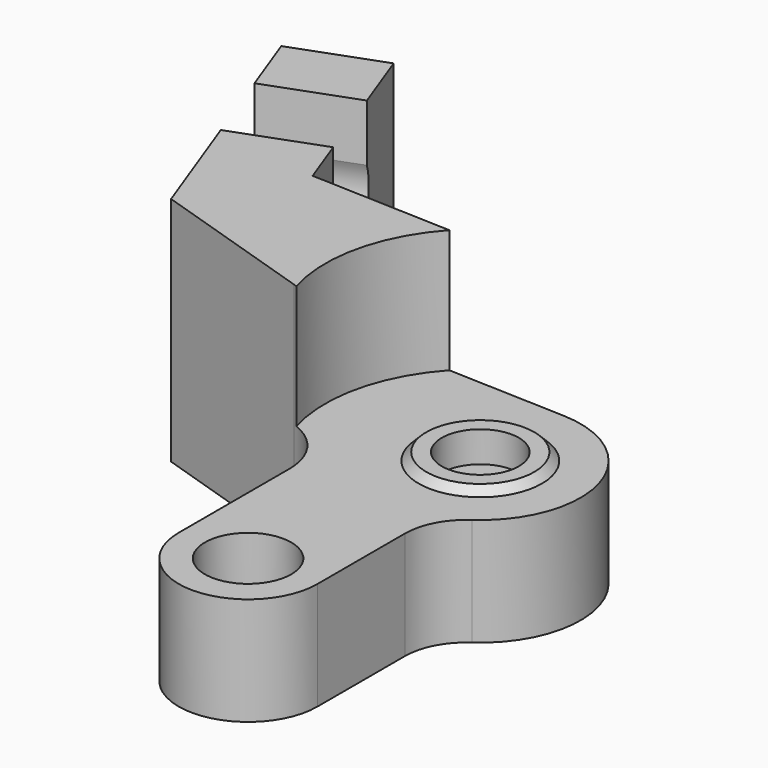
from build123d import *

# Parameters (mm, degrees)
F1_DEPTH       = 15
F3_DEPTH       = 8
F5_D           = 3.2
F5_CBORE_D     = 5.6
F5_CBORE_DEPTH = 3
F6_R           = 4.5
F7_DEPTH       = 5
F8_R           = 4
F9_DEPTH       = 0.5
F10_R          = 2.5
F11_DEPTH      = 2
F12_SIZE       = 0.49999
F14_DEPTH      = 6
F15_R          = 4


# Not quite as in the source:
# - a fillet or chamfer is up to 0.001 mm smaller than in the source, because OpenCascade refuses the exact size


with BuildPart() as f1:
    # F0 (on Top) → F1 (new body)
    with BuildSketch(Plane.XY):
        with BuildLine():
            Line((2, -15.7), (2, -6.1846584384))
            ThreePointArc((2, -6.1846584384), (6.437849506, 0.8967127402), (0.2337698218, 6.4957949221))
            Line((0.2337698218, 6.4957949221), (-16.5553616693, 7.1))
            Line((-16.5553616693, 7.1), (-21.0553616693, 19.2963109177))
            Line((-21.0553616693, 19.2963109177), (-26.6844282466, 17.2193878407))
            Line((-26.6844282466, 17.2193878407), (-20.5672701971, 0.6401075063))
            Line((-20.5672701971, 0.6401075063), (-9.8485109145, -2.7956722641))
            ThreePointArc((-9.8485109145, -2.7956722641), (-7.7878175435, -4.283505147), (-7, -6.7))
            Line((-7, -6.7), (-7, -15.7))
            ThreePointArc((-7, -15.7), (-2.5, -20.2), (2, -15.7))
        make_face()
    extrude(amount=F1_DEPTH)

    # F2 (on face) → F3 (cut)
    with BuildSketch(Plane.XY.offset(15)):
        with BuildLine():
            Line((2, -15.7), (2, -9.8489847192))
            ThreePointArc((2, -9.8489847192), (2.8265485956, 9.6443311347), (-7, -7.2112758927))
            Line((-7, -7.2112758927), (-7, -15.7))
            ThreePointArc((-7, -15.7), (-2.5, -20.2), (2, -15.7))
        make_face()
    extrude(amount=-F3_DEPTH, mode=Mode.SUBTRACT)

    # F5 (through all)
    with Locations(Plane.XY.offset(7)):
        with Locations((-2.5, -15.7)):
            CounterBoreHole(F5_D / 2, F5_CBORE_D / 2, F5_CBORE_DEPTH)

    # F6 (on face) → F7 (cut)
    with BuildSketch(Plane(origin=(0, 0, 0), x_dir=(1, 0, 0), z_dir=(0, 0, -1))):
        Circle(F6_R)
    extrude(amount=-F7_DEPTH, mode=Mode.SUBTRACT)

    # F8 (on face) → F9 (join)
    with BuildSketch(Plane.XY.offset(7)):
        Circle(F8_R)
    extrude(amount=F9_DEPTH)

    # F10 (on face) → F11 (cut)
    with BuildSketch(Plane.XY.offset(7.5)):
        Circle(F10_R)
    extrude(amount=-F11_DEPTH, mode=Mode.SUBTRACT)

    # F12 (size 0.5 in the source; OpenCascade refuses exactly that, so slightly less here)
    f12_edges = [f1.edges().sort_by_distance(p)[0] for p in [
        (-4, 0, 7.5),
    ]]
    chamfer(f12_edges, length=F12_SIZE)

    # F13 (on face) → F14 (cut, through all)
    with BuildSketch(Plane(origin=(-17.8949713968, -6.6026007232, 0), x_dir=(0.3461538462, -0.9381777629, 0), z_dir=(-0.9381777629, -0.3461538462, 0))):
        with BuildLine():
            Line((-15.6917642328, 15), (-21.0917642328, 15))
            Line((-21.0917642328, 15), (-21.0917642328, 11.3076696831))
            ThreePointArc((-21.0917642328, 11.3076696831), (-18.3917642328, 7), (-15.6917642328, 11.3076696831))
            Line((-15.6917642328, 11.3076696831), (-15.6917642328, 15))
        make_face()
    extrude(amount=-F14_DEPTH, mode=Mode.SUBTRACT)

    # F15
    f15_edges = [f1.edges().sort_by_distance(p)[0] for p in [
        (2, -6.184658, 3.5),
    ]]
    fillet(f15_edges, radius=F15_R)


solid = f1.part
